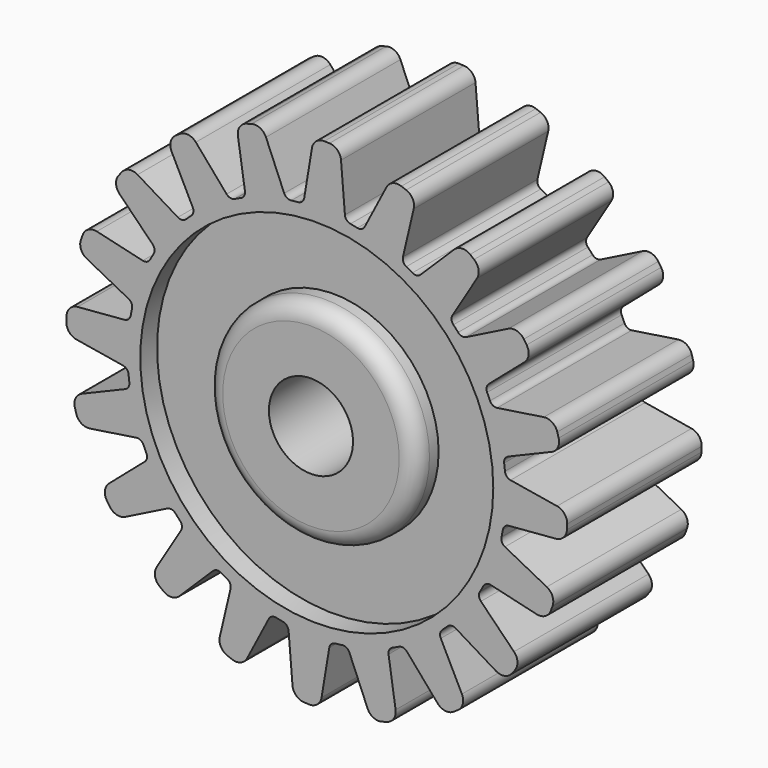
from build123d import *

# Parameters (mm, degrees)
F0_R            = 7.14375
F1_DEPTH        = 3.175
F3_DEPTH        = 6.35
F3_COPIES_COUNT = 20
F4_R            = 0.4572
F5_R            = 0.254
F6_R            = 6.6675
F7_DEPTH        = 0.79375
F8_R            = 3.96875
F9_DEPTH        = 1.0668
F10_R           = 0.635
F11_R           = 6.6675
F12_DEPTH       = 0.79375
F13_R           = 3.96875
F14_DEPTH       = 0.5334
F16_R           = 1.5875
F17_DEPTH       = 12.7


# Not quite as in the source:
# - a fillet or chamfer that OpenCascade refuses, or shapes differently, is made with other operations: its cross-section is extruded or revolved along the edge and cut away or added
# - a pattern or mirror of a feature is missing from the dataset's text; its kind, count and spacing are read off the source's solid


with BuildPart() as f1:
    # F0 (on Front) → F1 (new body, symmetric)
    with BuildSketch(Plane.XZ):
        Circle(F0_R)
    extrude(amount=F1_DEPTH, both=True)

    # F2 (on face) → F3 (join)
    with BuildSketch(Plane.XZ.offset(3.175)):
        Polygon((-0.1159478008, 9.4750692455), (-0.505261855, 7.1258595636), (1.0809328952, 7.0614975847), (0.8832299946, 9.4345262667), align=None)
    f3 = extrude(amount=-F3_DEPTH)

    # F3_copies: F3 ×20 about axis
    f3_copies_axis = Axis((0, 0, 0), (0, 1, 0))
    for i in range(1, F3_COPIES_COUNT):
        add(f3.rotate(f3_copies_axis, i * 360 / F3_COPIES_COUNT))

    # F4
    f4_edges = [f1.edges().sort_by_distance(p)[0] for p in [
        (-0.115948, 0, 9.475069),
        (0.88323, 0, 9.434526),
        (2.817685, 0, 9.047156),
        (9.245701, 0, 2.075427),
        (9.475069, 0, 0.115948),
        (9.434526, 0, -0.88323),
        (9.047156, 0, -2.817685),
        (8.699835, 0, -3.755431),
        (7.733644, 0, -5.475502),
        (7.113543, 0, -6.260023),
        (5.66311, 0, -7.59734),
        (4.830927, 0, -8.151842),
        (3.03823, 0, -8.975497),
        (2.075427, 0, -9.245701),
        (0.115948, 0, -9.475069),
        (-0.88323, 0, -9.434526),
        (-2.817685, 0, -9.047156),
        (-3.755431, 0, -8.699835),
        (-5.475502, 0, -7.733644),
        (-6.260023, 0, -7.113543),
        (-7.59734, 0, -5.66311),
        (-8.151842, 0, -4.830927),
        (-8.975497, 0, -3.03823),
        (-9.245701, 0, -2.075427),
        (-9.475069, 0, -0.115948),
        (-9.434526, 0, 0.88323),
        (-9.047156, 0, 2.817685),
        (-8.699835, 0, 3.755431),
        (-7.733644, 0, 5.475502),
        (-7.113543, 0, 6.260023),
        (-5.66311, 0, 7.59734),
        (-4.830927, 0, 8.151842),
        (3.755431, 0, 8.699835),
        (5.475502, 0, 7.733644),
        (6.260023, 0, 7.113543),
        (7.59734, 0, 5.66311),
        (8.151842, 0, 4.830927),
        (8.975497, 0, 3.03823),
        (-3.03823, 0, 8.975497),
        (-2.075427, 0, 9.245701),
    ]]
    fillet(f4_edges, radius=F4_R)

    # F5
    f5_edges = [f1.edges().sort_by_distance(p)[0] for p in [
        (-0.505262, 0, 7.12586),
        (1.080933, 0, 7.061498),
        (1.721479, 0, 6.93323),
        (-1.154094, 0, 7.04991),
        (3.210151, 0, 6.381857),
        (3.77971, 0, 6.061927),
        (-2.682544, 0, 6.620961),
        (-3.276151, 0, 6.348228),
        (5.025137, 0, 5.077515),
        (5.467956, 0, 4.597241),
        (-4.597241, 0, 5.467956),
        (-5.077515, 0, 5.025137),
        (6.348228, 0, 3.276151),
        (6.620961, 0, 2.682544),
        (-6.061927, 0, 3.77971),
        (-6.381857, 0, 3.210151),
        (7.04991, 0, 1.154094),
        (7.12586, 0, 0.505262),
        (-6.93323, 0, 1.721479),
        (-7.061498, 0, 1.080933),
        (7.061498, 0, -1.080933),
        (6.93323, 0, -1.721479),
        (-7.12586, 0, -0.505262),
        (-7.04991, 0, -1.154094),
        (6.381857, 0, -3.210151),
        (6.061927, 0, -3.77971),
        (-6.620961, 0, -2.682544),
        (-6.348228, 0, -3.276151),
        (5.077515, 0, -5.025137),
        (4.597241, 0, -5.467956),
        (-5.467956, 0, -4.597241),
        (-5.025137, 0, -5.077515),
        (3.276151, 0, -6.348228),
        (2.682544, 0, -6.620961),
        (-3.77971, 0, -6.061927),
        (-3.210151, 0, -6.381857),
        (1.154094, 0, -7.04991),
        (0.505262, 0, -7.12586),
        (-1.721479, 0, -6.93323),
        (-1.080933, 0, -7.061498),
    ]]
    fillet(f5_edges, radius=F5_R)

    # F6 (on face) → F7 (cut, symmetric)
    with BuildSketch(Plane.XZ.offset(3.175)):
        Circle(F6_R)
    extrude(amount=F7_DEPTH, both=True, mode=Mode.SUBTRACT)

    # F8 (on face) → F9 (join)
    with BuildSketch(Plane.XZ.offset(2.38125)):
        Circle(F8_R)
    extrude(amount=F9_DEPTH)

    # F10
    f10_edges = [f1.edges().sort_by_distance(p)[0] for p in [
        (-3.96875, -3.44805, 0),
    ]]
    fillet(f10_edges, radius=F10_R)

    # F11 (on face) → F12 (cut, symmetric)
    with BuildSketch(Plane(origin=(0, 3.175, 0), x_dir=(-1, 0, 0), z_dir=(0, 1, 0))):
        Circle(F11_R)
    extrude(amount=F12_DEPTH, both=True, mode=Mode.SUBTRACT)

    # F13 (on face) → F14 (join, symmetric)
    with BuildSketch(Plane(origin=(0, 2.38125, 0), x_dir=(-1, 0, 0), z_dir=(0, 1, 0))):
        Circle(F13_R)
    extrude(amount=F14_DEPTH, both=True)

    # F15: fillet of radius 0.635 on 1 edges, made by hand

    # F15_s1 → F15_t2 (revolve, cut)
    with BuildSketch(Plane.XY):
        with BuildLine():
            ThreePointArc((-3.96875, 2.38125), (-3.7534577302, 2.7632515922), (-3.3419306959, 2.91465))
            Line((-3.3419306959, 2.91465), (-3.96875, 2.91465))
            Line((-3.96875, 2.91465), (-3.96875, 2.38125))
        make_face()
    revolve(axis=Axis((0, 2.91465, 0), (0, 1, 0)), mode=Mode.SUBTRACT)

    # F16 (on face) → F17 (cut, symmetric)
    with BuildSketch(Plane(origin=(0, 2.91465, 0), x_dir=(-1, 0, 0), z_dir=(0, 1, 0))):
        Circle(F16_R)
    extrude(amount=F17_DEPTH, both=True, mode=Mode.SUBTRACT)


solid = f1.part
